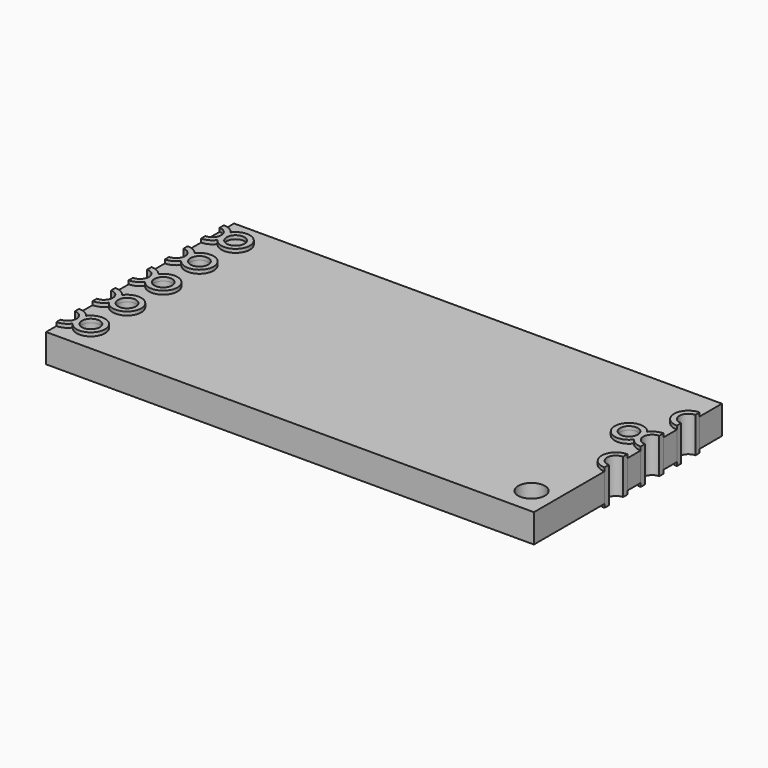
from build123d import *

# Parameters (mm, degrees)
F0_W          = 27.4
F0_H          = 13.2
F0_R          = 0.75
F1_DEPTH      = 1.6
F2_DEPTH      = 1.601
F4_DEPTH      = 0.2
F4_DEPTH_BACK = 1.8
F3_R          = 0.5
F5_DEPTH      = 1.801


# Not quite as in the source:
# - a feature names something its author has since deleted; it is built from what else it names


with BuildPart() as f1:
    # F0 (on Top) → F1 (new body)
    with BuildSketch(Plane.XY):
        Rectangle(F0_W, F0_H)
        with Locations((12.35, -5.08)):
            Circle(F0_R, mode=Mode.SUBTRACT)
        with Locations((12.35, -5.08)):
            Circle(F0_R)
    extrude(amount=-F1_DEPTH)

    # F0 (on Top) → F2 (cut, through all)
    with BuildSketch(Plane.XY):
        with Locations((12.35, -5.08)):
            Circle(F0_R)
    extrude(amount=-F2_DEPTH, mode=Mode.SUBTRACT)

    # F3 (on face) → F5 (cut, through all)
    with BuildSketch(Plane.XY):
        with Locations((-12.4, 2.54)):
            Circle(F3_R)
        with BuildLine():
            ThreePointArc((-13.7, 2.04), (-13.2, 2.54), (-13.7, 3.04))
            Line((-13.7, 3.04), (-13.7, 2.04))
        make_face()
        with Locations((-12.4, 0)):
            Circle(F3_R)
        with BuildLine():
            ThreePointArc((-13.7, -0.5), (-13.2, 0), (-13.7, 0.5))
            Line((-13.7, 0.5), (-13.7, -0.5))
        make_face()
        with Locations((-12.4, -2.54)):
            Circle(F3_R)
        with BuildLine():
            Line((-13.7, -2.04), (-13.7, -3.04))
            ThreePointArc((-13.7, -3.04), (-13.2, -2.54), (-13.7, -2.04))
        make_face()
        with Locations((-12.4, -5.08)):
            Circle(F3_R)
        with BuildLine():
            Line((-13.7, -4.58), (-13.7, -5.58))
            ThreePointArc((-13.7, -5.58), (-13.2, -5.08), (-13.7, -4.58))
        make_face()
        with BuildLine():
            Line((13.7, -1.34), (13.7, -0.34))
            ThreePointArc((13.7, -0.34), (13.2, -0.84), (13.7, -1.34))
        make_face()
        with BuildLine():
            Line((13.7, 3.74), (13.7, 4.74))
            ThreePointArc((13.7, 4.74), (13.2, 4.24), (13.7, 3.74))
        make_face()
        with BuildLine():
            Line((13.7, 1.2), (13.7, 2.2))
            ThreePointArc((13.7, 2.2), (13.2, 1.7), (13.7, 1.2))
        make_face()
        with Locations((12.4, 1.7)):
            Circle(F3_R)
    extrude(amount=-F5_DEPTH, mode=Mode.SUBTRACT)


with BuildPart() as f4:
    # F3 (on face) → F4 (new body, two sides)
    with BuildSketch(Plane.XY) as f4_sk:
        with BuildLine():
            Line((13.7, -0.34), (13.7, -0.04))
            ThreePointArc((13.7, -0.04), (12.9, -0.84), (13.7, -1.64))
            Line((13.7, -1.64), (13.7, -1.34))
            ThreePointArc((13.7, -1.34), (13.2, -0.84), (13.7, -0.34))
        make_face()
    extrude(amount=F4_DEPTH)
    extrude(f4_sk.sketch, amount=-F4_DEPTH_BACK)


with BuildPart() as f4b:
    # F3 (on face) → F4, piece 2 (new body, two sides)
    with BuildSketch(Plane.XY) as f4_2_sk:
        with BuildLine():
            Line((-13.7, -5.58), (-13.7, -5.88))
            ThreePointArc((-13.7, -5.88), (-13.3346886, -5.7917215615), (-13.05, -5.5463689527))
            ThreePointArc((-13.05, -5.5463689527), (-11.6, -5.08), (-13.05, -4.6136310473))
            ThreePointArc((-13.05, -4.6136310473), (-13.3346886, -4.3682784385), (-13.7, -4.28))
            Line((-13.7, -4.28), (-13.7, -4.58))
            ThreePointArc((-13.7, -4.58), (-13.2, -5.08), (-13.7, -5.58))
        make_face()
        with Locations((-12.4, -5.08)):
            Circle(F3_R, mode=Mode.SUBTRACT)
    extrude(amount=F4_DEPTH)
    extrude(f4_2_sk.sketch, amount=-F4_DEPTH_BACK)


with BuildPart() as f4c:
    # F3 (on face) → F4, piece 3 (new body, two sides)
    with BuildSketch(Plane.XY) as f4_3_sk:
        with BuildLine():
            ThreePointArc((-13.05, 5.5463689527), (-13.3346886, 5.7917215615), (-13.7, 5.88))
            Line((-13.7, 5.88), (-13.7, 5.58))
            ThreePointArc((-13.7, 5.58), (-13.2, 5.08), (-13.7, 4.58))
            Line((-13.7, 4.58), (-13.7, 4.28))
            ThreePointArc((-13.7, 4.28), (-13.3346886, 4.3682784385), (-13.05, 4.6136310473))
            ThreePointArc((-13.05, 4.6136310473), (-11.6, 5.08), (-13.05, 5.5463689527))
        make_face()
        with Locations((-12.4, 5.08)):
            Circle(F3_R, mode=Mode.SUBTRACT)
    extrude(amount=F4_DEPTH)
    extrude(f4_3_sk.sketch, amount=-F4_DEPTH_BACK)


with BuildPart() as f4d:
    # F3 (on face) → F4, piece 4 (new body, two sides)
    with BuildSketch(Plane.XY) as f4_4_sk:
        with BuildLine():
            ThreePointArc((-13.05, 3.0063689527), (-13.3346886, 3.2517215615), (-13.7, 3.34))
            Line((-13.7, 3.34), (-13.7, 3.04))
            ThreePointArc((-13.7, 3.04), (-13.2, 2.54), (-13.7, 2.04))
            Line((-13.7, 2.04), (-13.7, 1.74))
            ThreePointArc((-13.7, 1.74), (-13.3346886, 1.8282784385), (-13.05, 2.0736310473))
            ThreePointArc((-13.05, 2.0736310473), (-11.6, 2.54), (-13.05, 3.0063689527))
        make_face()
        with Locations((-12.4, 2.54)):
            Circle(F3_R, mode=Mode.SUBTRACT)
    extrude(amount=F4_DEPTH)
    extrude(f4_4_sk.sketch, amount=-F4_DEPTH_BACK)


with BuildPart() as f4e:
    # F3 (on face) → F4, piece 5 (new body, two sides)
    with BuildSketch(Plane.XY) as f4_5_sk:
        with BuildLine():
            ThreePointArc((-13.05, 0.4663689527), (-13.3346886, 0.7117215615), (-13.7, 0.8))
            Line((-13.7, 0.8), (-13.7, 0.5))
            ThreePointArc((-13.7, 0.5), (-13.2, 0), (-13.7, -0.5))
            Line((-13.7, -0.5), (-13.7, -0.8))
            ThreePointArc((-13.7, -0.8), (-13.3346886, -0.7117215615), (-13.05, -0.4663689527))
            ThreePointArc((-13.05, -0.4663689527), (-11.6, 0), (-13.05, 0.4663689527))
        make_face()
        with Locations((-12.4, 0)):
            Circle(F3_R, mode=Mode.SUBTRACT)
    extrude(amount=F4_DEPTH)
    extrude(f4_5_sk.sketch, amount=-F4_DEPTH_BACK)


with BuildPart() as f4f:
    # F3 (on face) → F4, piece 6 (new body, two sides)
    with BuildSketch(Plane.XY) as f4_6_sk:
        with BuildLine():
            Line((-13.7, -3.04), (-13.7, -3.34))
            ThreePointArc((-13.7, -3.34), (-13.3346886, -3.2517215615), (-13.05, -3.0063689527))
            ThreePointArc((-13.05, -3.0063689527), (-11.6, -2.54), (-13.05, -2.0736310473))
            ThreePointArc((-13.05, -2.0736310473), (-13.3346886, -1.8282784385), (-13.7, -1.74))
            Line((-13.7, -1.74), (-13.7, -2.04))
            ThreePointArc((-13.7, -2.04), (-13.2, -2.54), (-13.7, -3.04))
        make_face()
        with Locations((-12.4, -2.54)):
            Circle(F3_R, mode=Mode.SUBTRACT)
    extrude(amount=F4_DEPTH)
    extrude(f4_6_sk.sketch, amount=-F4_DEPTH_BACK)


with BuildPart() as f4g:
    # F3 (on face) → F4, piece 7 (new body, two sides)
    with BuildSketch(Plane.XY) as f4_7_sk:
        with BuildLine():
            ThreePointArc((13.7, 3.74), (13.2, 4.24), (13.7, 4.74))
            Line((13.7, 4.74), (13.7, 5.04))
            ThreePointArc((13.7, 5.04), (12.9, 4.24), (13.7, 3.44))
            Line((13.7, 3.44), (13.7, 3.74))
        make_face()
    extrude(amount=F4_DEPTH)
    extrude(f4_7_sk.sketch, amount=-F4_DEPTH_BACK)


with BuildPart() as f4h:
    # F3 (on face) → F4, piece 8 (new body, two sides)
    with BuildSketch(Plane.XY) as f4_8_sk:
        with BuildLine():
            Line((13.7, 2.2), (13.7, 2.5))
            ThreePointArc((13.7, 2.5), (13.3346886, 2.4117215615), (13.05, 2.1663689527))
            ThreePointArc((13.05, 2.1663689527), (11.6, 1.7), (13.05, 1.2336310473))
            ThreePointArc((13.05, 1.2336310473), (13.3346886, 0.9882784385), (13.7, 0.9))
            Line((13.7, 0.9), (13.7, 1.2))
            ThreePointArc((13.7, 1.2), (13.2, 1.7), (13.7, 2.2))
        make_face()
        with Locations((12.4, 1.7)):
            Circle(F3_R, mode=Mode.SUBTRACT)
    extrude(amount=F4_DEPTH)
    extrude(f4_8_sk.sketch, amount=-F4_DEPTH_BACK)


solid = Compound([f1.part, f4.part, f4b.part, f4c.part, f4d.part, f4e.part, f4f.part, f4g.part, f4h.part])
